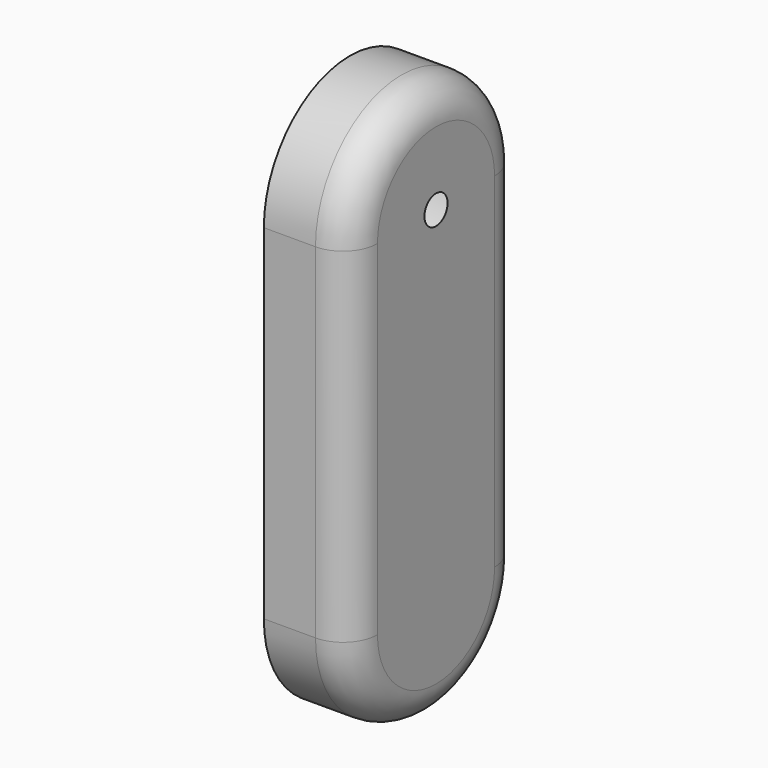
from build123d import *

# Parameters (mm, degrees)
F1_DEPTH = 12.7
F2_R     = 5.08
F4_D     = 25.4
F4_DEPTH = 6.35
F4_TIP   = 7.6309298617


# Not quite as in the source:
# - a feature names something its author has since deleted; it is built from what else it names


with BuildPart() as f1:
    # F0 (on Right) → F1 (new body)
    with BuildSketch(Plane.YZ):
        with BuildLine():
            ThreePointArc((-15.875, 0), (0, -15.875), (15.875, 0))
            ThreePointArc((15.875, 0), (0, 15.875), (-15.875, 0))
        make_face()
        with BuildLine():
            Line((15.875, -50.8), (15.875, 0))
            ThreePointArc((15.875, 0), (0, -15.875), (-15.875, 0))
            Line((-15.875, 0), (-15.875, -50.8))
            ThreePointArc((-15.875, -50.8), (0, -34.925), (15.875, -50.8))
        make_face()
        with BuildLine():
            ThreePointArc((-15.875, -50.8), (0, -66.675), (15.875, -50.8))
            ThreePointArc((15.875, -50.8), (0, -34.925), (-15.875, -50.8))
        make_face()
    extrude(amount=F1_DEPTH)

    # F2
    f2_edges = [f1.edges().sort_by_distance(p)[0] for p in [
        (12.7, 0, 15.875),
        (12.7, -15.875, -25.4),
        (12.7, 0, -66.675),
        (12.7, 15.875, -25.4),
    ]]
    fillet(f2_edges, radius=F2_R)

    # F4
    with Locations(Plane(origin=(0, 0, 0), x_dir=(0, -1, 0), z_dir=(-1, 0, 0))):
        with Locations((0, 0)):
            Hole(F4_D / 2, depth=F4_DEPTH)
            with Locations((0, 0, -(F4_DEPTH + F4_TIP / 2))):  # 118° drill point
                Cone(0, F4_D / 2, F4_TIP, mode=Mode.SUBTRACT)


solid = f1.part
